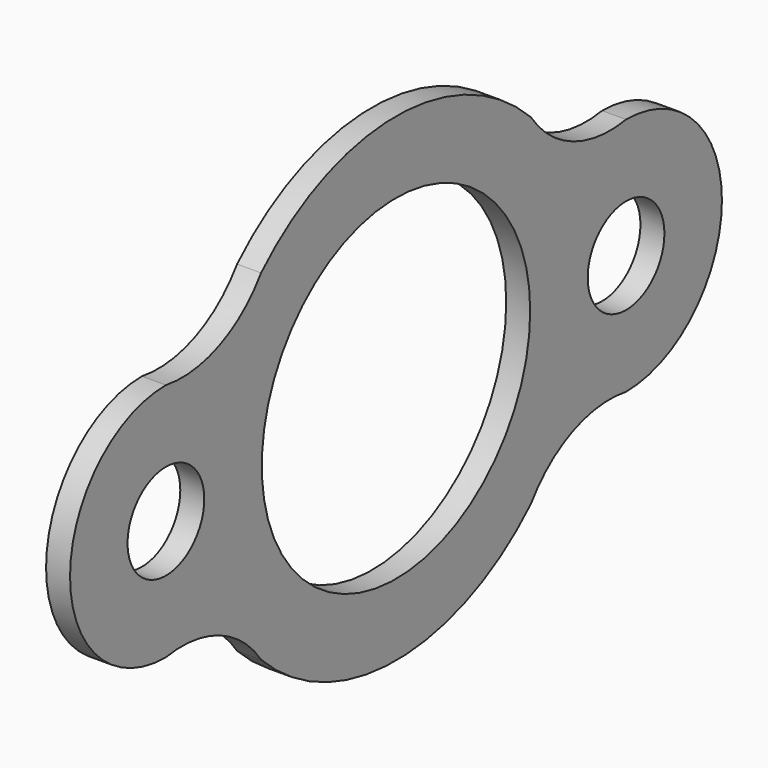
from build123d import *

# Parameters (mm, degrees)
F0_R     = 12.7
F0_R_2   = 44.45
F1_DEPTH = 6.35


# Not quite as in the source:
# - a length typed as a fraction of an inch, garbled in the dataset ("3 / 203.2 mm" for 3/8 in), is restored


with BuildPart() as f1:
    # F0 (on Right) → F1 (new body)
    with BuildSketch(Plane.YZ):
        with BuildLine():
            Line((44.8562400312, 44.8719321083), (44.6357637569, 45.1652365635))
            ThreePointArc((44.6357637569, 45.1652365635), (-0.039236718, 63.4999878778), (-44.6915449582, 45.1100411133))
            ThreePointArc((-44.6915449582, 45.1100411133), (-58.4915893115, 33.8212553621), (-76.2, 31.75))
            ThreePointArc((-76.2, 31.75), (-107.95, 0), (-76.2, -31.75))
            ThreePointArc((-76.2, -31.75), (-58.4915893115, -33.8212553621), (-44.6915449582, -45.1100411133))
            ThreePointArc((-44.6915449582, -45.1100411133), (0, -63.5), (44.6915449582, -45.1100411133))
            ThreePointArc((44.6915449582, -45.1100411133), (58.4915893115, -33.8212553621), (76.2, -31.75))
            ThreePointArc((76.2, -31.75), (107.95, 0), (76.2, 31.75))
            ThreePointArc((76.2, 31.75), (58.6249913094, 33.7650494266), (44.8562400312, 44.8719321083))
        make_face()
        with Locations((-76.2, 0)):
            Circle(F0_R, mode=Mode.SUBTRACT)
        Circle(F0_R_2, mode=Mode.SUBTRACT)
        with Locations((76.2, 0)):
            Circle(F0_R, mode=Mode.SUBTRACT)
    extrude(amount=F1_DEPTH)


solid = f1.part
